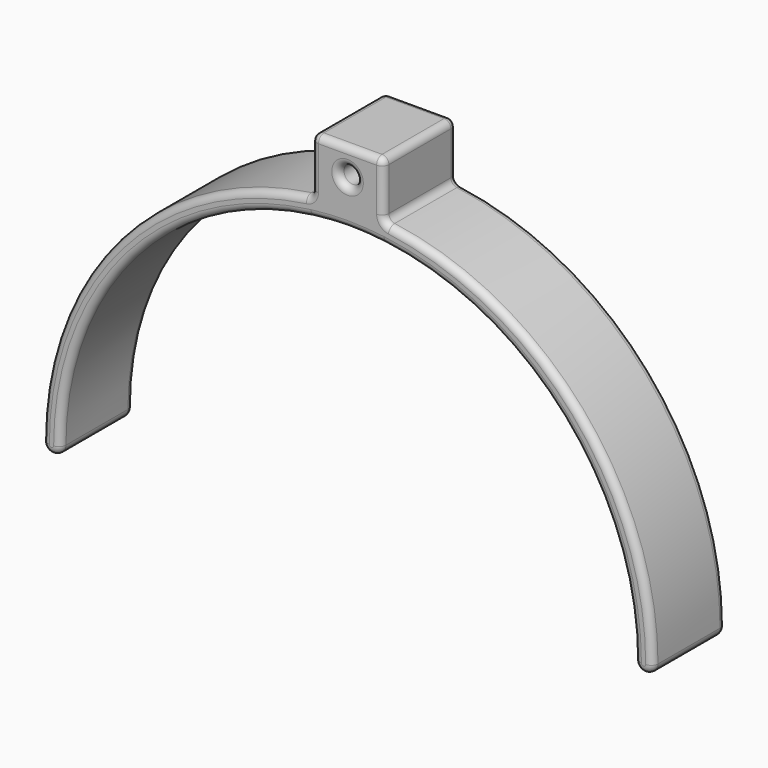
from build123d import *

# Parameters (mm, degrees)
F0_R     = 2.5
F1_DEPTH = 25.4
F2_R     = 1.905


with BuildPart() as f1:
    # F0 (on Front) → F1 (new body)
    with BuildSketch(Plane.XZ):
        with BuildLine():
            ThreePointArc((-85, 0), (-82.5, -2.5), (-80, 0))
            ThreePointArc((-80, 0), (-82.5, 2.5), (-85, 0))
        make_face()
        with BuildLine():
            ThreePointArc((-80, 0), (-60, 52.9150262213), (-10, 79.3725393319))
            Line((-10, 79.3725393319), (-10, 84.4097150807))
            ThreePointArc((-10, 84.4097150807), (-63.5413251357, 56.4579489532), (-85, 0))
            ThreePointArc((-85, 0), (-82.5, 2.5), (-80, 0))
        make_face()
        with BuildLine():
            ThreePointArc((-10, 84.4097150807), (0, 85), (10, 84.4097150807))
            Line((10, 84.4097150807), (10, 100))
            Line((10, 100), (-10, 100))
            Line((-10, 100), (-10, 84.4097150807))
        make_face()
        with Locations((0, 92.5)):
            Circle(F0_R, mode=Mode.SUBTRACT)
        with BuildLine():
            ThreePointArc((-10, 79.3725393319), (0, 80), (10, 79.3725393319))
            Line((10, 79.3725393319), (10, 84.4097150807))
            ThreePointArc((10, 84.4097150807), (0, 85), (-10, 84.4097150807))
            Line((-10, 84.4097150807), (-10, 79.3725393319))
        make_face()
        with BuildLine():
            ThreePointArc((10, 79.3725393319), (60, 52.9150262213), (80, 0))
            ThreePointArc((80, 0), (82.5, -2.5), (85, 0))
            ThreePointArc((85, 0), (63.5413251357, 56.4579489532), (10, 84.4097150807))
            Line((10, 84.4097150807), (10, 79.3725393319))
        make_face()
    extrude(amount=F1_DEPTH)

    # F2
    f2_edges = [f1.edges().sort_by_distance(p)[0] for p in [
        (85, -12.7, 0),
        (10, -12.7, 84.409715),
        (63.541325, 0, 56.457949),
        (63.541325, -25.4, 56.457949),
        (-82.5, 0, -2.5),
        (0, 0, 80),
        (82.5, 0, -2.5),
        (10, 0, 92.204858),
        (0, 0, 100),
        (-10, 0, 92.204858),
        (-63.541325, 0, 56.457949),
        (-2.5, 0, 92.5),
        (-2.5, -25.4, 92.5),
        (-10, -12.7, 100),
        (-10, -12.7, 84.409715),
        (-10, -25.4, 92.204858),
        (10, -12.7, 100),
        (0, -25.4, 100),
        (-82.5, -25.4, -2.5),
        (0, -25.4, 80),
        (82.5, -25.4, -2.5),
        (10, -25.4, 92.204858),
        (-63.541325, -25.4, 56.457949),
    ]]
    fillet(f2_edges, radius=F2_R)


solid = f1.part
